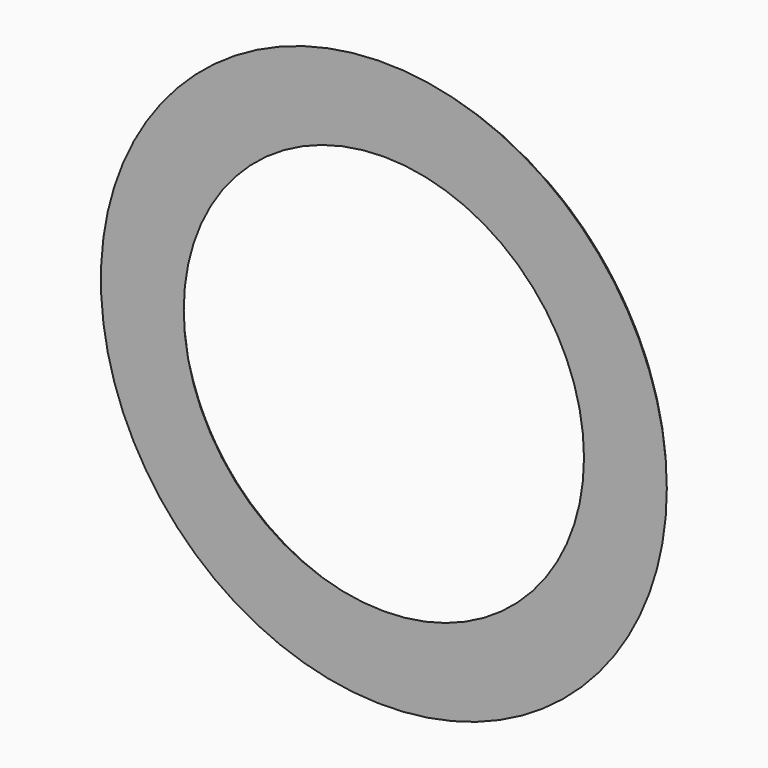
from build123d import *

# Parameters (mm, degrees)
F0_R     = 42.42
F0_R_2   = 30
F1_DEPTH = 3


# Not quite as in the source:
# - a fillet or chamfer that OpenCascade refuses, or shapes differently, is made with other operations: its cross-section is extruded or revolved along the edge and cut away or added


with BuildPart() as f1:
    # F0 (on Front) → F1 (new body)
    with BuildSketch(Plane.XZ):
        Circle(F0_R)
        Circle(F0_R_2, mode=Mode.SUBTRACT)
    extrude(amount=F1_DEPTH)

    # F2: fillet of radius 7.5 on 2 edges, made by hand

    # F2_s1 → F2_t2 (revolve, cut)
    with BuildSketch(Plane.XY):
        with BuildLine():
            ThreePointArc((30, -3), (32.6458980338, -0.7917960675), (36, 0))
            Line((36, 0), (30, 0))
            Line((30, 0), (30, -3))
        make_face()
    revolve(axis=Axis((0, 0, 0), (0, -1, 0)), mode=Mode.SUBTRACT)

    # F2_s3 → F2_t4 (revolve, cut)
    with BuildSketch(Plane.XY):
        with BuildLine():
            ThreePointArc((42.42, -3), (39.7741019662, -0.7917960675), (36.42, 0))
            Line((36.42, 0), (42.42, 0))
            Line((42.42, 0), (42.42, -3))
        make_face()
    revolve(axis=Axis((0, 0, 0), (0, -1, 0)), mode=Mode.SUBTRACT)


solid = f1.part
